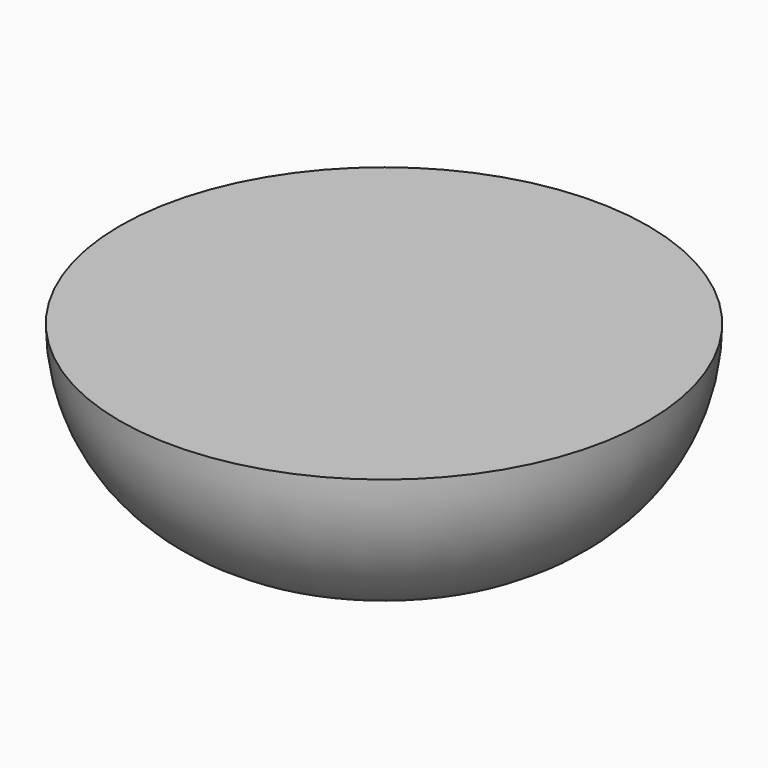
from build123d import *

# Parameters (mm, degrees)
F0_R     = 5
F1_DEPTH = 5
F0_R_2   = 7.5
F2_DEPTH = 5
F3_R     = 4.99999


# Not quite as in the source:
# - a fillet or chamfer is up to 0.001 mm smaller than in the source, because OpenCascade refuses the exact size


with BuildPart() as f1:
    # F0 (on Top) → F1 (new body)
    with BuildSketch(Plane.XY):
        Circle(F0_R)
    extrude(amount=F1_DEPTH)

    # F0 (on Top) → F2 (join)
    with BuildSketch(Plane.XY):
        Circle(F0_R_2)
        Circle(F0_R, mode=Mode.SUBTRACT)
    extrude(amount=F2_DEPTH)

    # F3 (radius 5 in the source; OpenCascade refuses exactly that, so slightly less here)
    f3_edges = [f1.edges().sort_by_distance(p)[0] for p in [
        (-7.5, 0, 0),
    ]]
    fillet(f3_edges, radius=F3_R)


solid = f1.part
